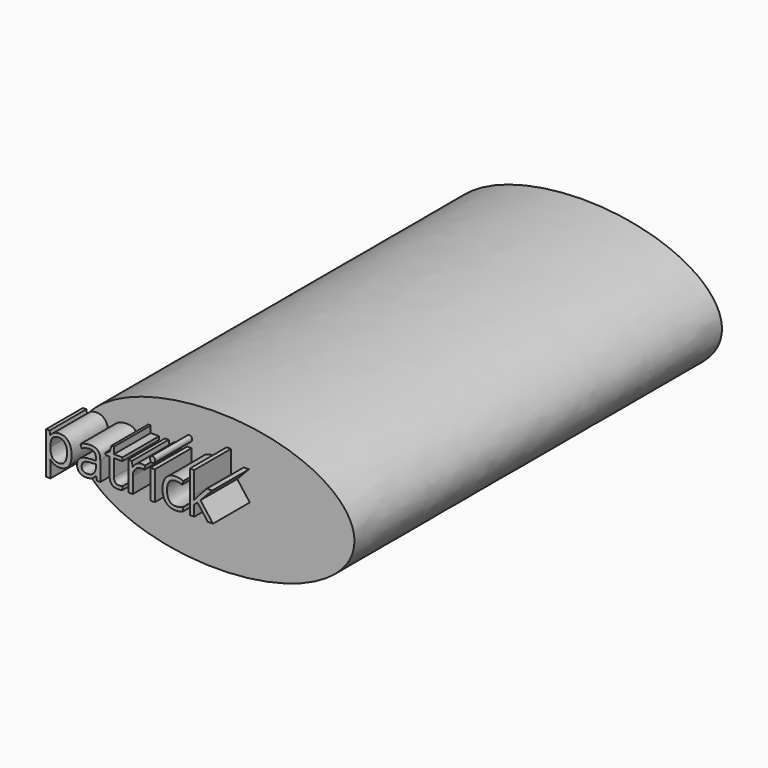
from build123d import *

# Parameters (mm, degrees)
F1_DEPTH     = 254
F2_TEXT_SIZE = 29.8952272
F3_DEPTH     = 25.4


# Not quite as in the source:
# - Text() gives the source's letters only with a copy of the font that has no kerning and outlines rounded to 1/6400 em; it was checked with that copy


with BuildPart() as f1:
    # F0 (on Front) → F1 (new body)
    with BuildSketch(Plane.XZ):
        with BuildLine():
            add(Edge.make_bspline(
                [(-76.3642266393, 0), (-76.3642266393, -66.0480758557), (38.1821133196, -33.0240379278), (152.7284532785, 0), (38.1821133196, 33.0240379278), (-76.3642266393, 66.0480758557), (-76.3642266393, 0)],
                knots=[0, 0, 0, 2.0943951024, 2.0943951024, 4.1887902048, 4.1887902048, 6.2831853072, 6.2831853072, 6.2831853072], degree=2, weights=[1, 0.5, 1, 0.5, 1, 0.5, 1]))
        make_face()
    extrude(amount=F1_DEPTH)

    # F2 (on face) → F3 (join)
    with BuildSketch(Plane.XZ.offset(254)):
        with Locations((-76.3642266393, 0)):
            Text('patrick', F2_TEXT_SIZE, font='Open Sans', text_align=(TextAlign.LEFT, TextAlign.BOTTOM))
    extrude(amount=F3_DEPTH)


solid = f1.part
